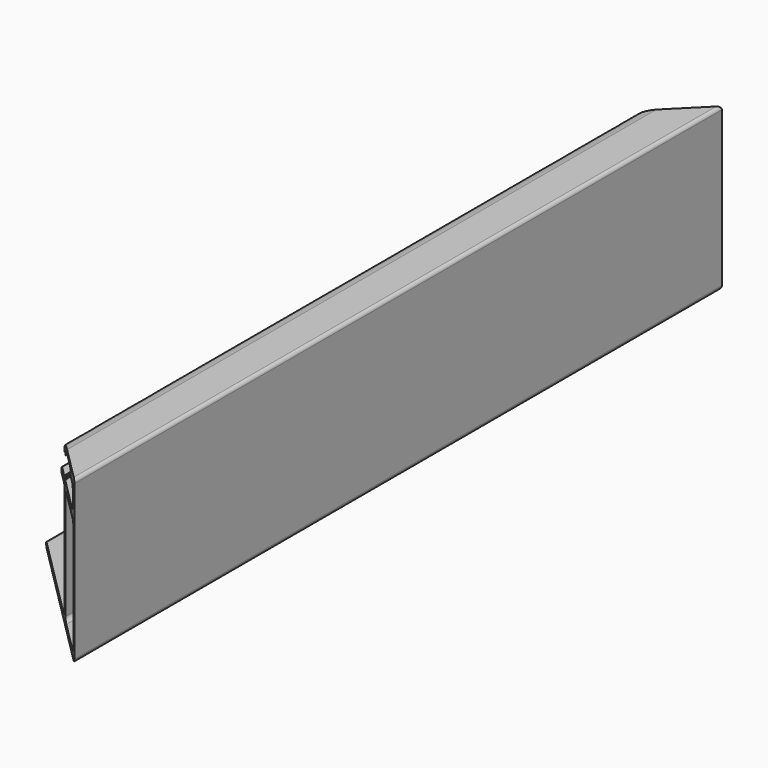
from build123d import *

# Parameters (mm, degrees)
F0_W        = 9.6591939426
F0_H        = 28.7
F1_DEPTH    = 200
F3_R        = 1
F4_R        = 1
F5_R        = 1
F6_R        = 0.3
F7_T1_DEPTH = 204
F8_R        = 1
F9_R        = 0.8
F10_R       = 0.5
F11_DEPTH   = 40.0010001


# Not quite as in the source:
# - a fillet or chamfer that OpenCascade refuses, or shapes differently, is made with other operations: its cross-section is extruded or revolved along the edge and cut away or added


with BuildPart() as f1:
    # F0 (on Front) → F1 (new body)
    with BuildSketch(Plane.XZ):
        with BuildLine():
            add(Edge.make_bspline(
                [(23, 38.132454922), (22.9909009473, 39.4079380262), (24.6147458735, 39.9568075433), (26.0023356814, 40)],
                knots=[0, 0, 0, 0, 3.5347881, 3.5347881, 3.5347881, 3.5347881], degree=3))
            Line((23, 38.132454922), (23, 37.5))
            Line((23, 37.5), (23.3642607927, 37.5))
            Line((23.3642607927, 37.5), (23.3642607927, 38.0080822861))
            Line((23.3642607927, 38.0080822861), (23.8452493811, 38.0080822861))
            Line((23.8452493811, 38.0080822861), (23.8452493811, 37.5))
            Line((23.8452493811, 37.5), (24.1986030313, 37.5))
            add(Edge.make_bspline(
                [(24.1986030313, 37.5), (23.7402990776, 39.8885678506), (29.4077517188, 38.843408227), (30.681502074, 39)],
                knots=[0, 0, 0, 0, 6.6541701209, 6.6541701209, 6.6541701209, 6.6541701209], degree=3))
            Line((30.681502074, 39), (30, 37.5))
            Line((30, 37.5), (33, 37.5))
            Line((33, 37.5), (33, 31.7))
            Line((33, 31.7), (23.6065152377, 31.7))
            Line((23.6065152377, 31.7), (23.6065152377, 31.5))
            Line((23.6065152377, 31.5), (23.2065152377, 31.5))
            Line((23.2065152377, 31.5), (23.2065152377, 31.7))
            Line((23.2065152377, 31.7), (22.7607861161, 31.7))
            Line((22.7607861161, 31.7), (22.7607861161, 31.5))
            Line((22.7607861161, 31.5), (22.3607861161, 31.5))
            Line((22.3607861161, 31.5), (22.3607861161, 31.7))
            Line((22.3607861161, 31.7), (19.7864715389, 31.7))
            Line((19.7864715389, 31.7), (19, 31.0823734798))
            Line((19, 31.0823734798), (19, 30.0495919195))
            ThreePointArc((19, 30.0495919195), (19.1617787134, 30.1431279745), (19.2819274904, 30))
            Line((19.2819274904, 30), (22.7408060574, 30))
            Line((22.7408060574, 30), (22.7408060574, 1.3))
            Line((22.7408060574, 1.3), (0, 1.3))
            Line((0, 1.3), (0, 0))
            Line((0, 0), (35, 0))
            Line((35, 0), (35, 40))
            Line((35, 40), (26.3559219739, 40))
            Line((26.3559219739, 40), (26.0023356814, 40))
        make_face()
        with Locations((28.8704030287, 15.65)):
            Rectangle(F0_W, F0_H, mode=Mode.SUBTRACT)
        with BuildLine():
            Line((23.3642607927, 37.5), (23, 37.5))
            ThreePointArc((23, 37.5), (23.1821303964, 37.3178696036), (23.3642607927, 37.5))
        make_face()
        with BuildLine():
            Line((24.1986030313, 37.5), (23.8452493811, 37.5))
            ThreePointArc((23.8452493811, 37.5), (24.0219262062, 37.3233231749), (24.1986030313, 37.5))
        make_face()
    extrude(amount=F1_DEPTH)

    # F3
    f3_edges = [f1.edges().sort_by_distance(p)[0] for p in [
        (33.7, -100, 30),
        (33.7, -100, 1.3),
        (24.040806, -100, 1.3),
        (24.040806, -100, 30),
    ]]
    fillet(f3_edges, radius=F3_R)

    # F4
    f4_edges = [f1.edges().sort_by_distance(p)[0] for p in [
        (22.740806, -100, 1.3),
    ]]
    fillet(f4_edges, radius=F4_R)

    # F5
    f5_edges = [f1.edges().sort_by_distance(p)[0] for p in [
        (33, -100, 31.7),
        (33, -100, 37.5),
    ]]
    fillet(f5_edges, radius=F5_R)

    # F6
    f6_edges = [f1.edges().sort_by_distance(p)[0] for p in [
        (30.681502, -100, 39),
    ]]
    fillet(f6_edges, radius=F6_R)

    # F7: fillet of radius 0.8 on 2 edges, made by hand

    # F7_s2 → F7_t1 (cut)
    with BuildSketch(Plane.XZ.offset(-2)):
        with BuildLine():
            ThreePointArc((0, 0.5), (0.2343145751, 1.0656854249), (0.8, 1.3))
            Line((0.8, 1.3), (0, 1.3))
            Line((0, 1.3), (0, 0.5))
        make_face()
        with BuildLine():
            ThreePointArc((0.8, 0), (0.2343145751, 0.2343145751), (0, 0.8))
            Line((0, 0.8), (0, 0))
            Line((0, 0), (0.8, 0))
        make_face()
    extrude(amount=F7_T1_DEPTH, mode=Mode.SUBTRACT)

    # F8
    f8_edges = [f1.edges().sort_by_distance(p)[0] for p in [
        (35, -100, 0),
    ]]
    fillet(f8_edges, radius=F8_R)

    # F9
    f9_edges = [f1.edges().sort_by_distance(p)[0] for p in [
        (35, -100, 40),
    ]]
    fillet(f9_edges, radius=F9_R)

    # F10
    f10_edges = [f1.edges().sort_by_distance(p)[0] for p in [
        (22.740806, -100, 30),
    ]]
    fillet(f10_edges, radius=F10_R)

    # F2 (on face) → F11 (cut, through all)
    with BuildSketch(Plane(origin=(0, 0, 0), x_dir=(1, 0, 0), z_dir=(0, 0, -1))):
        Polygon((0, 165), (35, 200), (0, 200), align=None)
        Polygon((0, 0), (35, 0), (0, 35), align=None)
    extrude(amount=-F11_DEPTH, mode=Mode.SUBTRACT)


solid = f1.part
